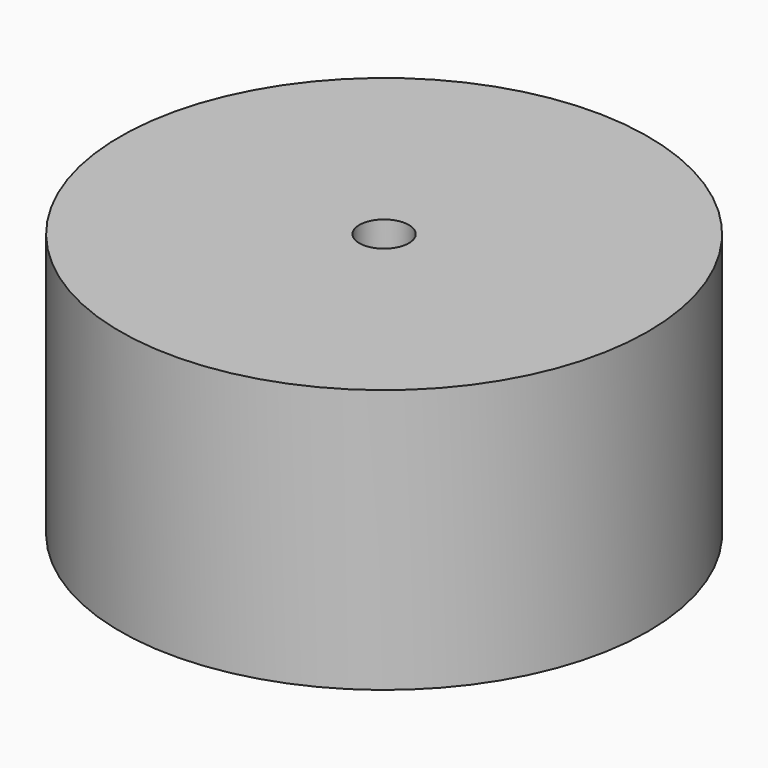
from build123d import *

# Parameters (mm, degrees)
F0_R     = 1.5
F0_R_2   = 0.75
F1_DEPTH = 7
F0_R_3   = 8
F0_R_4   = 7.5
F2_R     = 8
F2_R_2   = 1.5
F2_R_3   = 0.75
F3_DEPTH = 1


with BuildPart() as f1:
    # F0 (on Top) → F1 (new body)
    with BuildSketch(Plane.XY):
        Circle(F0_R)
        Circle(F0_R_2, mode=Mode.SUBTRACT)
    extrude(amount=F1_DEPTH)


with BuildPart() as f1b:
    # F0 (on Top) → F1, piece 2 (new body)
    with BuildSketch(Plane.XY):
        Circle(F0_R_3)
        Circle(F0_R_4, mode=Mode.SUBTRACT)
    extrude(amount=F1_DEPTH)

    # F2 (on face) → F3 (join)
    with BuildSketch(Plane.XY.offset(7)):
        Circle(F2_R)
        Circle(F2_R_2, mode=Mode.SUBTRACT)
        Circle(F2_R_2)
        Circle(F2_R_3, mode=Mode.SUBTRACT)
    extrude(amount=F3_DEPTH)


solid = Compound([f1.part, f1b.part])
